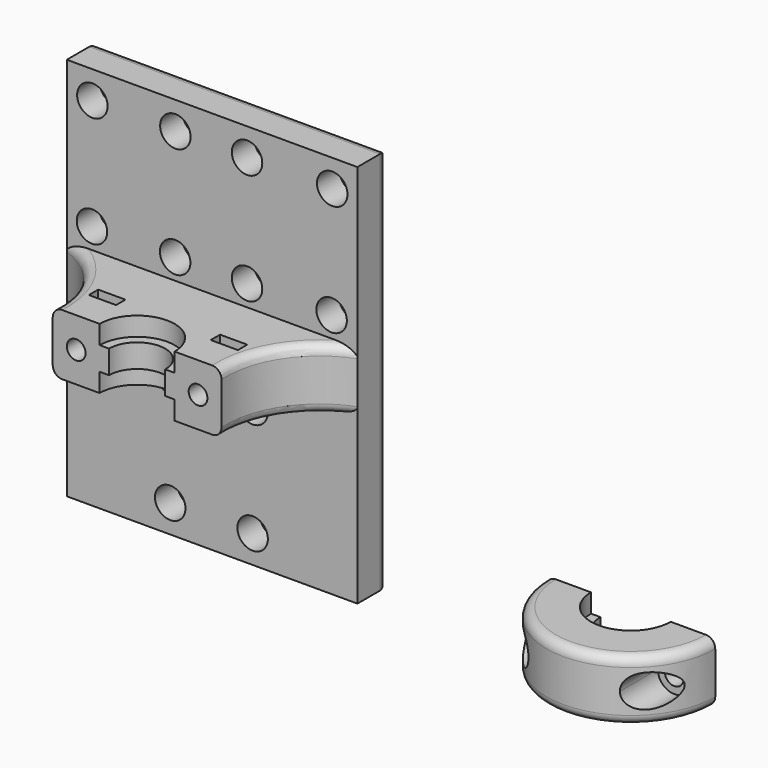
from build123d import *

# Parameters (mm, degrees)
F0_R          = 3.25
F1_DEPTH      = 8
F0_R_2        = 2
F2_DEPTH      = 2
F3_W          = 62
F3_H          = 13
F4_DEPTH      = 20
F6_DEPTH      = 25
F5_W          = 5.8
F5_H          = 2.5
F7_DEPTH      = 9
F8_DEPTH      = 25
F9_DEPTH      = 9
F10_DEPTH     = 4
F12_DEPTH     = 15
F14_DEPTH     = 15
F15_T1_DEPTH  = 72
F15_T3_DEPTH  = 92
F15_T8_ANGLE  = 101.8723701298
F15_T13_ANGLE = 101.8723701298
F15_T18_ANGLE = 101.8723701298
F15_T23_ANGLE = 101.8723701298
F17_DEPTH     = 13
F18_DEPTH     = 9
F19_DEPTH     = 4
F21_DEPTH     = 25
F22_DEPTH     = 5
F24_DEPTH     = 25
F25_DEPTH     = 5
F26_R         = 2
F27_DEPTH     = 9


# Not quite as in the source:
# - a fillet or chamfer that OpenCascade refuses, or shapes differently, is made with other operations: its cross-section is extruded or revolved along the edge and cut away or added
# - a feature names something its author has since deleted; it is built from what else it names


with BuildPart() as f1:
    # F0 (on Front) → F1 (new body)
    with BuildSketch(Plane.XZ):
        Polygon((-16, 0), (0, 0), (0, 48), (-30, 48), (-30, 82), (-32, 82), (-32, 48), (-62, 48), (-62, 0), (-46, 0), (-46, 34), (-16, 34), (-16, 31.7), (-16, 3.9), align=None)
        Polygon((-20.3, 0), (-16, 0), (-16, 3.9), (-16, 31.7), (-16, 34), (-46, 34), (-46, 0), (-42, 0), align=None)
        with Locations((-39.9336437008, 5.9503045419)):
            Circle(F0_R, mode=Mode.SUBTRACT)
        with Locations((-39.9147044088, 29.6257751592)):
            Circle(F0_R, mode=Mode.SUBTRACT)
        with Locations((-22.356529557, 5.9291128521)):
            Circle(F0_R, mode=Mode.SUBTRACT)
        with Locations((-22.3687138807, 29.6420210505)):
            Circle(F0_R, mode=Mode.SUBTRACT)
        Polygon((-30, 48), (0, 48), (0, 50.3), (0, 78.3), (0, 82), (-3.3, 82), (-25.3, 82), (-30, 82), align=None)
        with Locations((-23.55, 52.479400725)):
            Circle(F0_R, mode=Mode.SUBTRACT)
        with Locations((-5.5055998771, 52.4038018526)):
            Circle(F0_R, mode=Mode.SUBTRACT)
        with Locations((-23.55, 76.1129934432)):
            Circle(F0_R, mode=Mode.SUBTRACT)
        with Locations((-5.3714587349, 76.1748082815)):
            Circle(F0_R, mode=Mode.SUBTRACT)
        Polygon((-32, 48), (-32, 82), (-36.7, 82), (-58.7, 82), (-62, 82), (-62, 48), align=None)
        with Locations((-56.6326594642, 52.4275203692)):
            Circle(F0_R, mode=Mode.SUBTRACT)
        with Locations((-38.8890052369, 52.4363113403)):
            Circle(F0_R, mode=Mode.SUBTRACT)
        with Locations((-56.5488329259, 76.0989097772)):
            Circle(F0_R, mode=Mode.SUBTRACT)
        with Locations((-38.8392303967, 76.075045232)):
            Circle(F0_R, mode=Mode.SUBTRACT)
    extrude(amount=F1_DEPTH)

    # F0 (on Front) → F2 (join)
    with BuildSketch(Plane.XZ):
        with Locations((-56.5488329259, 76.0989097772)):
            Circle(F0_R)
        with Locations((-56.5488329259, 76.0989097772)):
            Circle(F0_R_2, mode=Mode.SUBTRACT)
        with Locations((-38.8392303967, 76.075045232)):
            Circle(F0_R)
        with Locations((-38.8392303967, 76.075045232)):
            Circle(F0_R_2, mode=Mode.SUBTRACT)
        with Locations((-23.55, 76.1129934432)):
            Circle(F0_R)
        with Locations((-23.55, 76.1129934432)):
            Circle(F0_R_2, mode=Mode.SUBTRACT)
        with Locations((-5.3714587349, 76.1748082815)):
            Circle(F0_R)
        with Locations((-5.3714587349, 76.1748082815)):
            Circle(F0_R_2, mode=Mode.SUBTRACT)
        with Locations((-5.5055998771, 52.4038018526)):
            Circle(F0_R)
        with Locations((-5.5055998771, 52.4038018526)):
            Circle(F0_R_2, mode=Mode.SUBTRACT)
        with Locations((-23.55, 52.479400725)):
            Circle(F0_R)
        with Locations((-23.55, 52.479400725)):
            Circle(F0_R_2, mode=Mode.SUBTRACT)
        with Locations((-38.8890052369, 52.4363113403)):
            Circle(F0_R)
        with Locations((-38.8890052369, 52.4363113403)):
            Circle(F0_R_2, mode=Mode.SUBTRACT)
        with Locations((-56.6326594642, 52.4275203692)):
            Circle(F0_R)
        with Locations((-56.6326594642, 52.4275203692)):
            Circle(F0_R_2, mode=Mode.SUBTRACT)
        with Locations((-39.9147044088, 29.6257751592)):
            Circle(F0_R)
        with Locations((-39.9147044088, 29.6257751592)):
            Circle(F0_R_2, mode=Mode.SUBTRACT)
        with Locations((-22.3687138807, 29.6420210505)):
            Circle(F0_R)
        with Locations((-22.3687138807, 29.6420210505)):
            Circle(F0_R_2, mode=Mode.SUBTRACT)
        with Locations((-22.356529557, 5.9291128521)):
            Circle(F0_R)
        with Locations((-22.356529557, 5.9291128521)):
            Circle(F0_R_2, mode=Mode.SUBTRACT)
        with Locations((-39.9336437008, 5.9503045419)):
            Circle(F0_R)
        with Locations((-39.9336437008, 5.9503045419)):
            Circle(F0_R_2, mode=Mode.SUBTRACT)
    extrude(amount=F2_DEPTH)

    # F3 (on face) → F4 (join)
    with BuildSketch(Plane.XZ.offset(8)):
        with Locations((-31, 41.5)):
            Rectangle(F3_W, F3_H)
    extrude(amount=F4_DEPTH)

    # F5 (on face) → F6 (cut)
    with BuildSketch(Plane.XY.offset(48)):
        with BuildLine():
            Line((-62, -8), (-62, -28))
            Line((-62, -28), (-49, -28))
            ThreePointArc((-49, -28), (-52.1919998258, -15.8497998867), (-62, -8))
        make_face()
        with BuildLine():
            Line((0, -28), (0, -8))
            ThreePointArc((0, -8), (-9.8080001742, -15.8497998867), (-13, -28))
            Line((-13, -28), (0, -28))
        make_face()
    extrude(amount=-F6_DEPTH, mode=Mode.SUBTRACT)

    # F5 (on face) → F7 (cut)
    with BuildSketch(Plane.XY.offset(48)):
        with Locations((-44, -19.75)):
            Rectangle(F5_W, F5_H)
    extrude(amount=-F7_DEPTH, mode=Mode.SUBTRACT)

    # F5 (on face) → F8 (cut)
    with BuildSketch(Plane.XY.offset(48)):
        with BuildLine():
            ThreePointArc((-25, -28), (-31, -22), (-37, -28))
            Line((-37, -28), (-25, -28))
        make_face()
        with BuildLine():
            ThreePointArc((-23, -28), (-31, -20), (-39, -28))
            Line((-39, -28), (-37, -28))
            ThreePointArc((-37, -28), (-31, -22), (-25, -28))
            Line((-25, -28), (-23, -28))
        make_face()
    extrude(amount=-F8_DEPTH, mode=Mode.SUBTRACT)

    # F5 (on face) → F9 (join)
    with BuildSketch(Plane.XY.offset(48)):
        with BuildLine():
            ThreePointArc((-23, -28), (-31, -20), (-39, -28))
            Line((-39, -28), (-37, -28))
            ThreePointArc((-37, -28), (-31, -22), (-25, -28))
            Line((-25, -28), (-23, -28))
        make_face()
    extrude(amount=-F9_DEPTH)

    # F5 (on face) → F10 (cut)
    with BuildSketch(Plane.XY.offset(48)):
        with BuildLine():
            ThreePointArc((-23, -28), (-31, -20), (-39, -28))
            Line((-39, -28), (-37, -28))
            ThreePointArc((-37, -28), (-31, -22), (-25, -28))
            Line((-25, -28), (-23, -28))
        make_face()
    extrude(amount=-F10_DEPTH, mode=Mode.SUBTRACT)

    # F11 (on face) → F12 (cut)
    with BuildSketch(Plane.XZ.offset(28)):
        with BuildLine():
            ThreePointArc((-44, 43.5), (-45.4142135624, 40.0857864376), (-42, 41.5))
            ThreePointArc((-42, 41.5), (-42.5857864376, 42.9142135624), (-44, 43.5))
        make_face()
    extrude(amount=-F12_DEPTH, mode=Mode.SUBTRACT)

    # F13 (on face) → F14 (cut)
    with BuildSketch(Plane.XZ.offset(28)):
        with BuildLine():
            ThreePointArc((-18, 43.5), (-19.4142135624, 40.0857864376), (-16, 41.5))
            ThreePointArc((-16, 41.5), (-16.5857864376, 42.9142135624), (-18, 43.5))
        make_face()
    extrude(amount=-F14_DEPTH, mode=Mode.SUBTRACT)

    # F15: fillet of radius 2 on 8 edges, made by hand

    # F15_s2 → F15_t1 (cut)
    with BuildSketch(Plane.YZ.offset(-67)):
        with BuildLine():
            ThreePointArc((0, 80), (-0.5857864376, 81.4142135624), (-2, 82))
            Line((-2, 82), (0, 82))
            Line((0, 82), (0, 80))
        make_face()
        with BuildLine():
            ThreePointArc((0, 2), (-0.5857864376, 0.5857864376), (-2, 0))
            Line((-2, 0), (0, 0))
            Line((0, 0), (0, 2))
        make_face()
    extrude(amount=F15_T1_DEPTH, mode=Mode.SUBTRACT)

    # F15_s4 → F15_t3 (cut)
    with BuildSketch(Plane.XY.offset(-5)):
        with BuildLine():
            ThreePointArc((-60, 0), (-61.4142135624, -0.5857864376), (-62, -2))
            Line((-62, -2), (-62, 0))
            Line((-62, 0), (-60, 0))
        make_face()
        with BuildLine():
            ThreePointArc((0, -2), (-0.5857864376, -0.5857864376), (-2, 0))
            Line((-2, 0), (0, 0))
            Line((0, 0), (0, -2))
        make_face()
    extrude(amount=F15_T3_DEPTH, mode=Mode.SUBTRACT)


with BuildPart() as f15_tool6:
    # F15_s7 → F15_t8 (revolve)
    with BuildSketch(Plane(origin=(4.0847901889, 0.4322083918, 0), x_dir=(0, 0, 1), z_dir=(0.994448775, 0.1052218317, 0))):
        with BuildLine():
            ThreePointArc((46, 7.3335097526), (47.4142135624, 6.747723315), (48, 5.3335097526))
            Line((48, 5.3335097526), (48, 7.3335097526))
            Line((48, 7.3335097526), (46, 7.3335097526))
        make_face()
    revolve(axis=Axis((6.9608721518, -26.7495668986, 48), (0, 0, 1)), revolution_arc=F15_T8_ANGLE)

    split(bisect_by=Plane.XZ.offset(8), keep=Keep.TOP)


with BuildPart() as f1_1:
    add(f1.part)

    # F15_t5: cut F15_tool6
    add(f15_tool6.part, mode=Mode.SUBTRACT)


with BuildPart() as f15_tool11:
    # F15_s12 → F15_t13 (revolve)
    with BuildSketch(Plane(origin=(4.0847901889, 0.4322083918, 0), x_dir=(0, 0, 1), z_dir=(0.994448775, 0.1052218317, 0))):
        with BuildLine():
            ThreePointArc((37, 7.3335097526), (35.5857864376, 6.747723315), (35, 5.3335097526))
            Line((35, 5.3335097526), (35, 7.3335097526))
            Line((35, 7.3335097526), (37, 7.3335097526))
        make_face()
    revolve(axis=Axis((6.9608721518, -26.7495668986, 35), (0, 0, 1)), revolution_arc=F15_T13_ANGLE)

    split(bisect_by=Plane.XZ.offset(8), keep=Keep.TOP)


with BuildPart() as f1_2:
    add(f1_1.part)

    # F15_t10: cut F15_tool11
    add(f15_tool11.part, mode=Mode.SUBTRACT)


with BuildPart() as f15_tool16:
    # F15_s17 → F15_t18 (revolve)
    with BuildSketch(Plane(origin=(-14.3516223114, -44.4008396076, 0), x_dir=(0, 0, 1), z_dir=(-0.3075611855, -0.951528306, 0))):
        with BuildLine():
            ThreePointArc((48, 35.391093354), (47.4142135624, 36.8053069164), (46, 37.391093354))
            Line((46, 37.391093354), (48, 37.391093354))
            Line((48, 37.391093354), (48, 35.391093354))
        make_face()
    revolve(axis=Axis((-68.9608721518, -26.7495668986, 48), (0, 0, 1)), revolution_arc=F15_T18_ANGLE)

    split(bisect_by=Plane.XZ.offset(8), keep=Keep.TOP)


with BuildPart() as f1_3:
    add(f1_2.part)

    # F15_t15: cut F15_tool16
    add(f15_tool16.part, mode=Mode.SUBTRACT)


with BuildPart() as f15_tool21:
    # F15_s22 → F15_t23 (revolve)
    with BuildSketch(Plane(origin=(-14.3516223114, -44.4008396076, 0), x_dir=(0, 0, 1), z_dir=(-0.3075611855, -0.951528306, 0))):
        with BuildLine():
            ThreePointArc((35, 35.391093354), (35.5857864376, 36.8053069164), (37, 37.391093354))
            Line((37, 37.391093354), (35, 37.391093354))
            Line((35, 37.391093354), (35, 35.391093354))
        make_face()
    revolve(axis=Axis((-68.9608721518, -26.7495668986, 35), (0, 0, 1)), revolution_arc=F15_T23_ANGLE)

    split(bisect_by=Plane.XZ.offset(8), keep=Keep.TOP)


with BuildPart() as f1_4:
    add(f1_3.part)

    # F15_t20: cut F15_tool21
    add(f15_tool21.part, mode=Mode.SUBTRACT)

    # F5 (on face) → F27 (cut)
    with BuildSketch(Plane.XY.offset(48)):
        with Locations((-18, -19.75)):
            Rectangle(F5_W, F5_H)
    extrude(amount=-F27_DEPTH, mode=Mode.SUBTRACT)


with BuildPart() as f17:
    # F16 (on Top) → F17 (new body)
    with BuildSketch(Plane.XY):
        with BuildLine():
            Line((43.4464648766, 0), (33.9464648766, 0))
            ThreePointArc((33.9464648766, 0), (51.9464648766, -18), (69.9464648766, 0))
            Line((69.9464648766, 0), (60.4464648766, 0))
            ThreePointArc((60.4464648766, 0), (51.9464648766, -8.5), (43.4464648766, 0))
        make_face()
    extrude(amount=F17_DEPTH)

    # F16 (on Top) → F18 (join)
    with BuildSketch(Plane.XY):
        with BuildLine():
            Line((45.4464648766, 0), (43.4464648766, 0))
            ThreePointArc((43.4464648766, 0), (51.9464648766, -8.5), (60.4464648766, 0))
            Line((60.4464648766, 0), (58.4464648766, 0))
            ThreePointArc((58.4464648766, 0), (51.9464648766, -6.5), (45.4464648766, 0))
        make_face()
    extrude(amount=F18_DEPTH)

    # F16 (on Top) → F19 (cut)
    with BuildSketch(Plane.XY):
        with BuildLine():
            Line((45.4464648766, 0), (43.4464648766, 0))
            ThreePointArc((43.4464648766, 0), (51.9464648766, -8.5), (60.4464648766, 0))
            Line((60.4464648766, 0), (58.4464648766, 0))
            ThreePointArc((58.4464648766, 0), (51.9464648766, -6.5), (45.4464648766, 0))
        make_face()
    extrude(amount=F19_DEPTH, mode=Mode.SUBTRACT)

    # F20 (on face) → F21 (cut)
    with BuildSketch(Plane(origin=(0, 0, 0), x_dir=(-1, 0, 0), z_dir=(0, 1, 0))):
        with BuildLine():
            ThreePointArc((-61.6964648766, 6.5), (-62.7215911425, 8.9748737342), (-65.1964648766, 10))
            ThreePointArc((-65.1964648766, 10), (-67.6713386108, 4.0251262658), (-61.6964648766, 6.5))
        make_face()
        with BuildLine():
            ThreePointArc((-63.1964648766, 6.5), (-66.610678439, 5.0857864376), (-65.1964648766, 8.5))
            ThreePointArc((-65.1964648766, 8.5), (-63.7822513143, 7.9142135624), (-63.1964648766, 6.5))
        make_face(mode=Mode.SUBTRACT)
        with BuildLine():
            ThreePointArc((-63.1964648766, 6.5), (-63.7822513143, 7.9142135624), (-65.1964648766, 8.5))
            ThreePointArc((-65.1964648766, 8.5), (-66.610678439, 5.0857864376), (-63.1964648766, 6.5))
        make_face()
    extrude(amount=-F21_DEPTH, mode=Mode.SUBTRACT)

    # F20 (on face) → F22 (join)
    with BuildSketch(Plane(origin=(0, 0, 0), x_dir=(-1, 0, 0), z_dir=(0, 1, 0))):
        with BuildLine():
            ThreePointArc((-61.6964648766, 6.5), (-62.7215911425, 8.9748737342), (-65.1964648766, 10))
            ThreePointArc((-65.1964648766, 10), (-67.6713386108, 4.0251262658), (-61.6964648766, 6.5))
        make_face()
        with BuildLine():
            ThreePointArc((-63.1964648766, 6.5), (-66.610678439, 5.0857864376), (-65.1964648766, 8.5))
            ThreePointArc((-65.1964648766, 8.5), (-63.7822513143, 7.9142135624), (-63.1964648766, 6.5))
        make_face(mode=Mode.SUBTRACT)
    extrude(amount=-F22_DEPTH)

    # F23 (on face) → F24 (cut)
    with BuildSketch(Plane(origin=(0, 0, 0), x_dir=(-1, 0, 0), z_dir=(0, 1, 0))):
        with BuildLine():
            ThreePointArc((-35.1964648766, 6.5), (-36.2215911425, 8.9748737342), (-38.6964648766, 10))
            ThreePointArc((-38.6964648766, 10), (-41.1713386108, 4.0251262658), (-35.1964648766, 6.5))
        make_face()
        with BuildLine():
            ThreePointArc((-36.6964648766, 6.5), (-40.110678439, 5.0857864376), (-38.6964648766, 8.5))
            ThreePointArc((-38.6964648766, 8.5), (-37.2822513143, 7.9142135624), (-36.6964648766, 6.5))
        make_face(mode=Mode.SUBTRACT)
        with BuildLine():
            ThreePointArc((-36.6964648766, 6.5), (-37.2822513143, 7.9142135624), (-38.6964648766, 8.5))
            ThreePointArc((-38.6964648766, 8.5), (-40.110678439, 5.0857864376), (-36.6964648766, 6.5))
        make_face()
    extrude(amount=-F24_DEPTH, mode=Mode.SUBTRACT)

    # F23 (on face) → F25 (join)
    with BuildSketch(Plane(origin=(0, 0, 0), x_dir=(-1, 0, 0), z_dir=(0, 1, 0))):
        with BuildLine():
            ThreePointArc((-35.1964648766, 6.5), (-36.2215911425, 8.9748737342), (-38.6964648766, 10))
            ThreePointArc((-38.6964648766, 10), (-41.1713386108, 4.0251262658), (-35.1964648766, 6.5))
        make_face()
        with BuildLine():
            ThreePointArc((-36.6964648766, 6.5), (-40.110678439, 5.0857864376), (-38.6964648766, 8.5))
            ThreePointArc((-38.6964648766, 8.5), (-37.2822513143, 7.9142135624), (-36.6964648766, 6.5))
        make_face(mode=Mode.SUBTRACT)
    extrude(amount=-F25_DEPTH)

    # F26
    f26_edges = [f17.edges().sort_by_distance(p)[0] for p in [
        (51.946465, -18, 13),
        (51.946465, -18, 0),
    ]]
    fillet(f26_edges, radius=F26_R)


solid = Compound([f1_4.part, f17.part])
